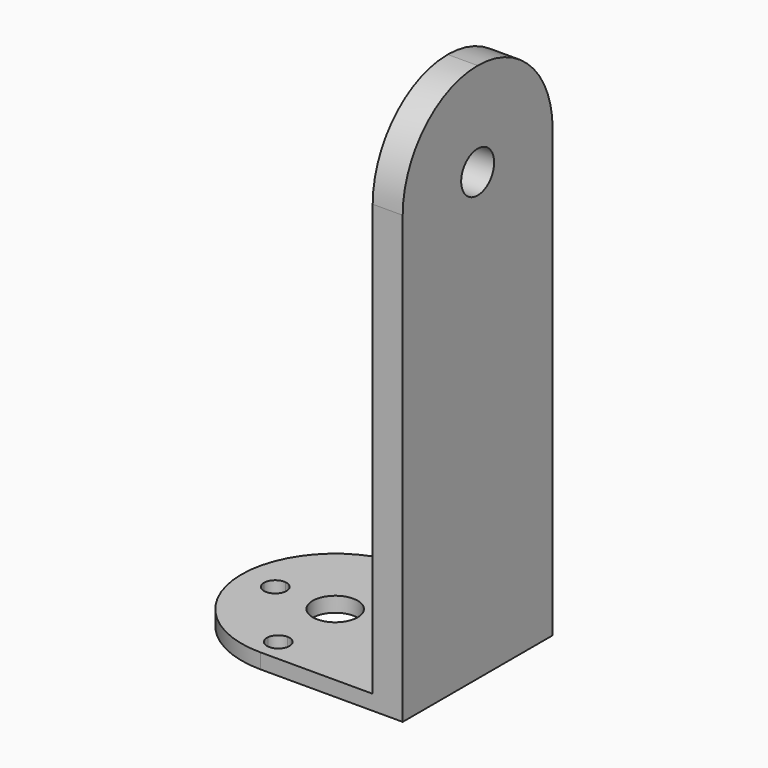
from build123d import *

# Parameters (mm, degrees)
F0_R     = 3
F1_DEPTH = 2
F2_W     = 4
F2_H     = 25
F3_DEPTH = 70
F4_R     = 2.75
F5_DEPTH = 31.501
F6_R     = 12.49999


# Not quite as in the source:
# - a fillet or chamfer is up to 0.001 mm smaller than in the source, because OpenCascade refuses the exact size
# - a feature names something its author has since deleted; it is built from what else it names


with BuildPart() as f1:
    # F0 (on Top) → F1 (new body)
    with BuildSketch(Plane.XY):
        with BuildLine():
            ThreePointArc((0, -12.5), (8.8388347648, -8.8388347648), (12.5, 0))
            ThreePointArc((12.5, 0), (8.8388347648, 8.8388347648), (0, 12.5))
            ThreePointArc((0, 12.5), (-12.5, 0), (0, -12.5))
        make_face()
        with BuildLine():
            ThreePointArc((1.4953181783, 9.3815789474), (7.2268777039, 6.1662175321), (9.5, 0))
            ThreePointArc((9.5, 0), (7.2268777039, -6.1662175321), (1.4953181783, -9.3815789474))
            ThreePointArc((1.4953181783, -9.3815789474), (1.4988290876, -9.4407432173), (1.5, -9.5))
            ThreePointArc((1.5, -9.5), (-0.0592567827, -10.9988290876), (-1.4953181783, -9.3815789474))
            ThreePointArc((-1.4953181783, -9.3815789474), (-7.2268777039, -6.1662175321), (-9.5, 0))
            ThreePointArc((-9.5, 0), (-7.2268777039, 6.1662175321), (-1.4953181783, 9.3815789474))
            ThreePointArc((-1.4953181783, 9.3815789474), (-0.0592567827, 10.9988290876), (1.5, 9.5))
            ThreePointArc((1.5, 9.5), (1.4988290876, 9.4407432173), (1.4953181783, 9.3815789474))
        make_face(mode=Mode.SUBTRACT)
        with BuildLine():
            ThreePointArc((0, 12.5), (8.8388347648, 8.8388347648), (12.5, 0))
            ThreePointArc((12.5, 0), (8.8388347648, -8.8388347648), (0, -12.5))
            Line((0, -12.5), (19, -12.5))
            Line((19, -12.5), (19, 12.5))
            Line((19, 12.5), (0, 12.5))
        make_face()
        with BuildLine():
            ThreePointArc((7.859375, -1.4933936552), (6.5, 0), (7.859375, 1.4933936552))
            ThreePointArc((7.859375, 1.4933936552), (5.1016100823, 6.1622702446), (1.34e-08, 8))
            ThreePointArc((1.34e-08, 8), (-5.101610072, 6.1622702532), (-7.859375, 1.4933936552))
            ThreePointArc((-7.859375, 1.4933936552), (-6.8907350407, 1.0097184013), (-6.5, 0))
            ThreePointArc((-6.5, 0), (-6.8907350407, -1.0097184013), (-7.859375, -1.4933936552))
            ThreePointArc((-7.859375, -1.4933936552), (-5.1016100771, -6.1622702489), (0, -8))
            ThreePointArc((0, -8), (5.1016100771, -6.1622702489), (7.859375, -1.4933936552))
        make_face()
        Circle(F0_R, mode=Mode.SUBTRACT)
        with BuildLine():
            ThreePointArc((7.859375, 1.4933936552), (9.0097184013, 1.1092649593), (9.5, 0))
            ThreePointArc((9.5, 0), (7.2268777039, 6.1662175321), (1.4953181783, 9.3815789474))
            ThreePointArc((1.4953181783, 9.3815789474), (1.0179313437, 8.3982669201), (1.34e-08, 8))
            ThreePointArc((1.34e-08, 8), (5.1016100823, 6.1622702446), (7.859375, 1.4933936552))
        make_face()
        with BuildLine():
            ThreePointArc((1.4953181783, -9.3815789474), (7.2268777039, -6.1662175321), (9.5, 0))
            ThreePointArc((9.5, 0), (9.0097184013, -1.1092649593), (7.859375, -1.4933936552))
            ThreePointArc((7.859375, -1.4933936552), (5.1016100771, -6.1622702489), (0, -8))
            ThreePointArc((0, -8), (1.0179313388, -8.3982669155), (1.4953181783, -9.3815789474))
        make_face()
        with BuildLine():
            ThreePointArc((1.34e-08, 8), (-1.0179313339, 8.3982669109), (-1.4953181783, 9.3815789474))
            ThreePointArc((-1.4953181783, 9.3815789474), (-7.2268777039, 6.1662175321), (-9.5, 0))
            ThreePointArc((-9.5, 0), (-9.0097184013, 1.1092649593), (-7.859375, 1.4933936552))
            ThreePointArc((-7.859375, 1.4933936552), (-5.101610072, 6.1622702532), (1.34e-08, 8))
        make_face()
        with BuildLine():
            ThreePointArc((-9.5, 0), (-7.2268777039, -6.1662175321), (-1.4953181783, -9.3815789474))
            ThreePointArc((-1.4953181783, -9.3815789474), (-1.0179313388, -8.3982669155), (0, -8))
            ThreePointArc((0, -8), (-5.1016100771, -6.1622702489), (-7.859375, -1.4933936552))
            ThreePointArc((-7.859375, -1.4933936552), (-9.0097184013, -1.1092649593), (-9.5, 0))
        make_face()
    extrude(amount=F1_DEPTH)

    # F2 (on face) → F3 (join)
    with BuildSketch(Plane.XY.offset(2)):
        with Locations((17, 0)):
            Rectangle(F2_W, F2_H)
    extrude(amount=F3_DEPTH)

    # F4 (on face) → F5 (cut, through all)
    with BuildSketch(Plane.YZ.offset(19)):
        with Locations((0, 59.5)):
            Circle(F4_R)
    extrude(amount=-F5_DEPTH, mode=Mode.SUBTRACT)

    # F6 (radius 12.5 in the source; OpenCascade refuses exactly that, so slightly less here)
    f6_edges = [f1.edges().sort_by_distance(p)[0] for p in [
        (17, -12.5, 72),
        (17, 12.5, 72),
    ]]
    fillet(f6_edges, radius=F6_R)


solid = f1.part
